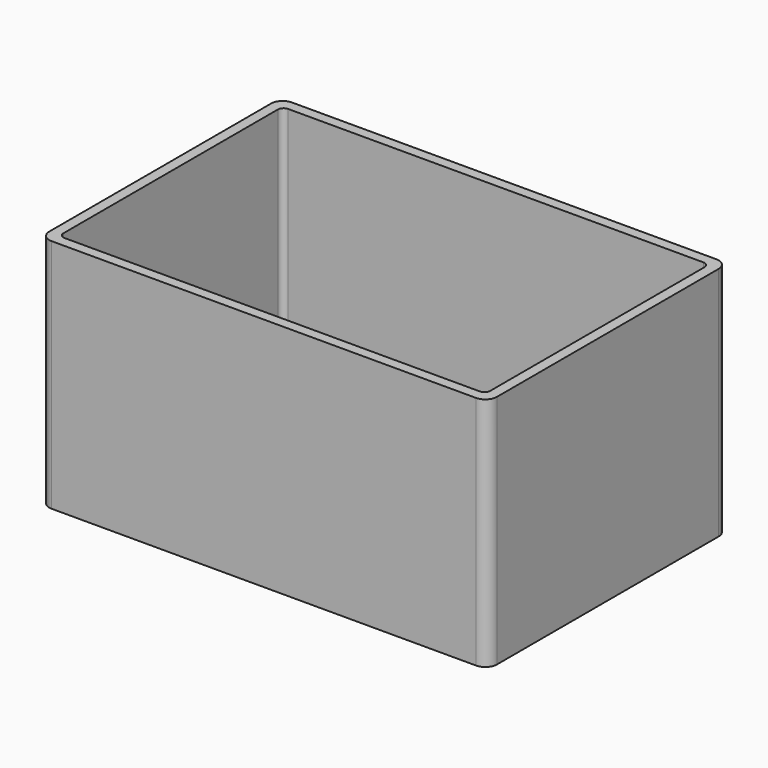
from build123d import *

# Parameters (mm, degrees)
F1_DEPTH = 40.64
F3_DEPTH = 38.608
F5_DEPTH = 4.7752
F6_R     = 1.35255
F7_DEPTH = 4.7752


# Not quite as in the source:
# - a feature names something its author has since deleted; it is built from what else it names


with BuildPart() as f1:
    # F0 (on Top) → F1 (new body)
    with BuildSketch(Plane.XY):
        with BuildLine():
            ThreePointArc((0, 2), (0.5857864376, 0.5857864376), (2, 0))
            Line((2, 0), (75.216, 0))
            ThreePointArc((75.216, 0), (76.6302135624, 0.5857864376), (77.216, 2))
            Line((77.216, 2), (77.216, 49.816))
            ThreePointArc((77.216, 49.816), (76.6302135624, 51.2302135624), (75.216, 51.816))
            Line((75.216, 51.816), (2, 51.816))
            ThreePointArc((2, 51.816), (0.5857864376, 51.2302135624), (0, 49.816))
            Line((0, 49.816), (0, 2))
        make_face()
    extrude(amount=F1_DEPTH)

    # F2 (on face) → F3 (cut)
    with BuildSketch(Plane.XY.offset(40.64)):
        with BuildLine():
            Line((74.416, 50.016), (2.8, 50.016))
            ThreePointArc((2.8, 50.016), (2.0928932188, 49.7231067812), (1.8, 49.016))
            Line((1.8, 49.016), (1.8, 2.8))
            ThreePointArc((1.8, 2.8), (2.0928932188, 2.0928932188), (2.8, 1.8))
            Line((2.8, 1.8), (74.416, 1.8))
            ThreePointArc((74.416, 1.8), (75.1231067812, 2.0928932188), (75.416, 2.8))
            Line((75.416, 2.8), (75.416, 49.016))
            ThreePointArc((75.416, 49.016), (75.1231067812, 49.7231067812), (74.416, 50.016))
        make_face()
    extrude(amount=-F3_DEPTH, mode=Mode.SUBTRACT)

    # F4 (on face) → F5 (join)
    with BuildSketch(Plane(origin=(0, 0, 0), x_dir=(1, 0, 0), z_dir=(0, 0, -1))):
        with BuildLine():
            ThreePointArc((77.216, -2), (76.6302135624, -0.5857864376), (75.216, 0))
            Line((75.216, 0), (71.406, 0))
            Line((71.406, 0), (71.406, -2))
            ThreePointArc((71.406, -2), (72.5219231637, -4.6940768363), (75.216, -5.81))
            Line((75.216, -5.81), (77.216, -5.81))
            Line((77.216, -5.81), (77.216, -2))
        make_face()
        with BuildLine():
            Line((71.406, -49.816), (71.406, -51.816))
            Line((71.406, -51.816), (75.216, -51.816))
            ThreePointArc((75.216, -51.816), (76.6302135624, -51.2302135624), (77.216, -49.816))
            Line((77.216, -49.816), (77.216, -46.006))
            Line((77.216, -46.006), (75.216, -46.006))
            ThreePointArc((75.216, -46.006), (72.5219231637, -47.1219231637), (71.406, -49.816))
        make_face()
        with BuildLine():
            ThreePointArc((5.81, -49.816), (4.6940768363, -47.1219231637), (2, -46.006))
            Line((2, -46.006), (0, -46.006))
            Line((0, -46.006), (0, -49.816))
            ThreePointArc((0, -49.816), (0.5857864376, -51.2302135624), (2, -51.816))
            Line((2, -51.816), (5.81, -51.816))
            Line((5.81, -51.816), (5.81, -49.816))
        make_face()
        with BuildLine():
            Line((5.81, 0), (2, 0))
            ThreePointArc((2, 0), (0.5857864376, -0.5857864376), (0, -2))
            Line((0, -2), (0, -5.81))
            Line((0, -5.81), (2, -5.81))
            ThreePointArc((2, -5.81), (4.6940768363, -4.6940768363), (5.81, -2))
            Line((5.81, -2), (5.81, 0))
        make_face()
    extrude(amount=-F5_DEPTH)

    # F6 (on face) → F7 (cut, through all)
    with BuildSketch(Plane(origin=(0, 0, 0), x_dir=(1, 0, 0), z_dir=(0, 0, -1))):
        with Locations((73.8658709242, -3.3501290758)):
            Circle(F6_R)
        with Locations((3.3501290758, -3.3501290758)):
            Circle(F6_R)
        with Locations((3.3501290758, -48.4658709242)):
            Circle(F6_R)
        with Locations((73.8658709242, -48.4658709242)):
            Circle(F6_R)
    extrude(amount=-F7_DEPTH, mode=Mode.SUBTRACT)


solid = f1.part
